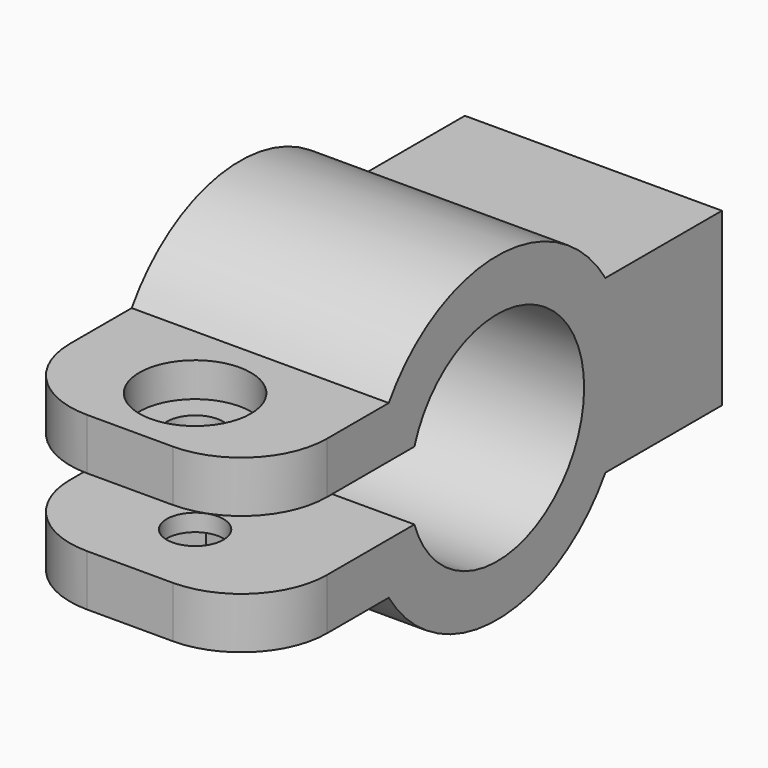
from build123d import *
from build123d import SkipClean  # not in build123d's __all__

# Parameters (mm, degrees)
F0_W           = 15
F0_H           = 10
F1_DEPTH       = 8.5
F3_DEPTH       = 7.5
F5_D           = 3.3
F5_CBORE_D     = 6.5
F5_CBORE_DEPTH = 2
F7_DEPTH       = 2
F8_R           = 5
F10_DEPTH      = 2
F11_T3_DEPTH   = 6.6704632943
F11_S4_R       = 2.6
F11_T5_DEPTH   = 5
F11_T8_DEPTH   = 6.6704632943
F11_S9_R       = 2.6
F11_T10_DEPTH  = 5
F11_T13_ANGLE  = 75.9597448897
F11_T16_ANGLE  = 75.9597448897
F11_T19_ANGLE  = 104.0402551103
F11_T22_ANGLE  = 104.0402551103


# Not quite as in the source:
# - a fillet or chamfer that OpenCascade refuses, or shapes differently, is made with other operations: its cross-section is extruded or revolved along the edge and cut away or added


with BuildPart() as f1:
    # F0 (on Front) → F1 (new body)
    with BuildSketch(Plane.XZ):
        Rectangle(F0_W, F0_H)
        with BuildLine():
            ThreePointArc((-2.0493901532, -1.6), (-2.6, 0), (-2.0493901532, 1.6))
            Line((-2.0493901532, 1.6), (2.0493901532, 1.6))
            ThreePointArc((2.0493901532, 1.6), (2.6, 0), (2.0493901532, -1.6))
            Line((2.0493901532, -1.6), (-2.0493901532, -1.6))
        make_face(mode=Mode.SUBTRACT)
    extrude(amount=-F1_DEPTH)

    # F2 (on Right) → F3 (join, symmetric)
    with BuildSketch(Plane.YZ):
        with BuildLine():
            ThreePointArc((-13.9276061789, 2), (-1.5507910996, 0), (-13.9276061789, -2))
            Line((-13.9276061789, -2), (-25.3015821993, -2))
            Line((-25.3015821993, -2), (-25.3015821993, -5))
            Line((-25.3015821993, -5), (-15.8015821993, -5))
            ThreePointArc((-15.8015821993, -5), (-7.9007910996, -9.35), (0, -5))
            Line((0, -5), (0, 5))
            ThreePointArc((0, 5), (-7.9007910996, 9.35), (-15.8015821993, 5))
            Line((-15.8015821993, 5), (-25.3015821993, 5))
            Line((-25.3015821993, 5), (-25.3015821993, 2))
            Line((-25.3015821993, 2), (-13.9276061789, 2))
        make_face()
    extrude(amount=F3_DEPTH, both=True)

    # F5 (through all)
    with Locations(Plane.XY.offset(5)):
        with Locations((0, -20.5515821993)):
            CounterBoreHole(F5_D / 2, F5_CBORE_D / 2, F5_CBORE_DEPTH)

    # F6 (on face) → F7 (cut)
    with BuildSketch(Plane(origin=(0, 0, -5), x_dir=(1, 0, 0), z_dir=(0, 0, -1))):
        Polygon((-1.6454482672, 17.7015821993), (1.6454482672, 17.7015821993), (3.2908965344, 20.5515821993), (1.6454482672, 23.4015821993), (-1.6454482672, 23.4015821993), (-3.2908965344, 20.5515821993), align=None)
    extrude(amount=-F7_DEPTH, mode=Mode.SUBTRACT)

    # F8
    f8_edges = [f1.edges().sort_by_distance(p)[0] for p in [
        (7.5, -25.301582, 3.5),
        (-7.5, -25.301582, 3.5),
        (-7.5, -25.301582, -3.5),
        (7.5, -25.301582, -3.5),
    ]]
    fillet(f8_edges, radius=F8_R)

    # F9 (on face) → F10 (cut)
    with BuildSketch(Plane(origin=(0, 8.5, 0), x_dir=(-1, 0, 0), z_dir=(0, 1, 0))):
        with BuildLine():
            Line((-2.0493901532, 1.6), (2.0493901532, 1.6))
            ThreePointArc((2.0493901532, 1.6), (0, 2.6), (-2.0493901532, 1.6))
        make_face()
        with BuildLine():
            ThreePointArc((-2.0493901532, -1.6), (0, -2.6), (2.0493901532, -1.6))
            Line((2.0493901532, -1.6), (-2.0493901532, -1.6))
        make_face()
    with SkipClean():  # cleaning this boolean's faces spoils the solid; the shape is the same uncleaned
        extrude(amount=-F10_DEPTH, mode=Mode.SUBTRACT)

    # F11: chamfer of 0.5 on 6 edges, made by hand


with BuildPart() as f11_tool1:
    # F11_s2 → F11_t3 (new body)
    with BuildSketch(Plane.YZ.offset(3.3352316472)):
        Polygon((6, 1.6), (6.5, 2.1), (6.5, 1.6), align=None)
    extrude(amount=-F11_T3_DEPTH)

    # F11_s4 → F11_t5 (intersect, symmetric)
    with BuildSketch(Plane.XZ.offset(-6.2)):
        Circle(F11_S4_R)
    extrude(amount=F11_T5_DEPTH, both=True, mode=Mode.INTERSECT)


with BuildPart() as f11_tool6:
    # F11_s7 → F11_t8 (new body)
    with BuildSketch(Plane.YZ.offset(-3.3352316472)):
        Polygon((6, -1.6), (6.5, -2.1), (6.5, -1.6), align=None)
    extrude(amount=F11_T8_DEPTH)

    # F11_s9 → F11_t10 (intersect, symmetric)
    with BuildSketch(Plane.XZ.offset(-6.2)):
        Circle(F11_S9_R)
    extrude(amount=F11_T10_DEPTH, both=True, mode=Mode.INTERSECT)


with BuildPart() as f11_tool11:
    # F11_s12 → F11_t13 (revolve)
    with BuildSketch(Plane(origin=(0, 0, 0), x_dir=(0, 1, 0), z_dir=(0.6153846154, 0, -0.788226982))):
        Polygon((8.5, -3.1), (8, -2.6), (8.5, -2.6), align=None)
    revolve(axis=Axis((0, 8.5, 0), (0, 1, 0)), revolution_arc=F11_T13_ANGLE)


with BuildPart() as f11_tool14:
    # F11_s15 → F11_t16 (revolve)
    with BuildSketch(Plane(origin=(0, 0, 0), x_dir=(0, 1, 0), z_dir=(-0.6153846154, 0, 0.788226982))):
        Polygon((8.5, -3.1), (8, -2.6), (8.5, -2.6), align=None)
    revolve(axis=Axis((0, 8.5, 0), (0, 1, 0)), revolution_arc=F11_T16_ANGLE)


with BuildPart() as f11_tool17:
    # F11_s18 → F11_t19 (revolve)
    with BuildSketch(Plane(origin=(0, 0, 0), x_dir=(0, 1, 0), z_dir=(-0.6153846154, 0, -0.788226982))):
        Polygon((8.5, -3.1), (8, -2.6), (8.5, -2.6), align=None)
    revolve(axis=Axis((0, 8.5, 0), (0, 1, 0)), revolution_arc=F11_T19_ANGLE)


with BuildPart() as f11_tool20:
    # F11_s21 → F11_t22 (revolve)
    with BuildSketch(Plane(origin=(0, 0, 0), x_dir=(0, 1, 0), z_dir=(0.6153846154, 0, 0.788226982))):
        Polygon((8.5, -3.1), (8, -2.6), (8.5, -2.6), align=None)
    revolve(axis=Axis((0, 8.5, 0), (0, 1, 0)), revolution_arc=F11_T22_ANGLE)


with BuildPart() as f1_1:
    add(f1.part, clean=False)

    # F11_t23: cut F11_tool1, F11_tool6, F11_tool11, F11_tool14, F11_tool17, F11_tool20
    add([f11_tool1.part, f11_tool6.part, f11_tool11.part, f11_tool14.part, f11_tool17.part, f11_tool20.part], mode=Mode.SUBTRACT)


solid = f1_1.part
